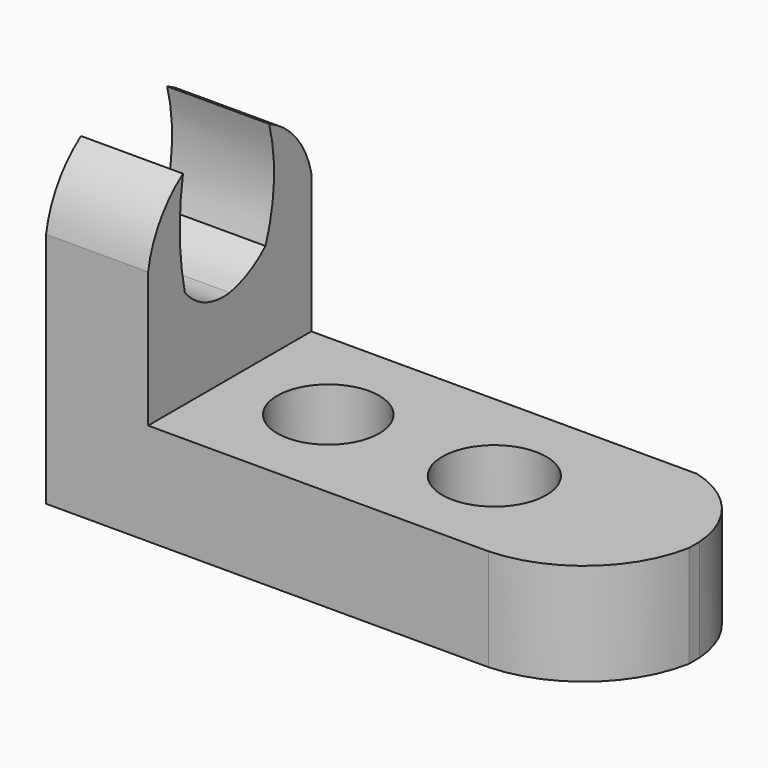
from build123d import *

# Parameters (mm, degrees)
F1_DEPTH = 25.4
F3_DEPTH = 25.4
F5_DEPTH = 25.4
F7_DEPTH = 25.4
F8_R     = 6.3524650116
F8_R_2   = 6.4782695501
F9_DEPTH = 25.4


with BuildPart() as f1:
    # F0 (on Front) → F1 (new body)
    with BuildSketch(Plane.XZ):
        Polygon((0, 38.1), (0, 0), (69.85, 0), (69.85, 12.7), (12.7, 12.7), (12.7, 38.1), align=None)
    extrude(amount=F1_DEPTH)

    # F2 (on face) → F3 (cut)
    with BuildSketch(Plane.XY.offset(12.7)):
        with BuildLine():
            ThreePointArc((69.85, -12.7), (64.6936030033, -21.620488158), (55.1082585024, -25.4))
            Line((55.1082585024, -25.4), (69.85, -25.4))
            Line((69.85, -25.4), (69.85, -12.7))
        make_face()
        with BuildLine():
            ThreePointArc((60.7121499118, 0), (67.063378566, -4.0558500097), (69.85, -11.0574759425))
            Line((69.85, -11.0574759425), (69.85, 0))
            Line((69.85, 0), (60.7121499118, 0))
        make_face()
    extrude(amount=-F3_DEPTH, mode=Mode.SUBTRACT)

    # F4 (on face) → F5 (cut)
    with BuildSketch(Plane.YZ.offset(12.7)):
        with BuildLine():
            ThreePointArc((-12.7, 22.1061483026), (-9.7123568594, 23.1357247682), (-7.1310154162, 24.958556518))
            ThreePointArc((-7.1310154162, 24.958556518), (-5.8144018077, 31.4845054838), (-6.5605342388, 38.1))
            Line((-6.5605342388, 38.1), (-19.9668444693, 38.1))
            ThreePointArc((-19.9668444693, 38.1), (-20.4652180352, 31.5153652578), (-19.6816045791, 24.958556518))
            ThreePointArc((-19.6816045791, 24.958556518), (-16.5691552263, 22.6062890993), (-12.7, 22.1061483026))
        make_face()
    extrude(amount=-F5_DEPTH, mode=Mode.SUBTRACT)

    # F6 (on face) → F7 (cut)
    with BuildSketch(Plane.YZ.offset(12.7)):
        with BuildLine():
            ThreePointArc((-25.4, 29.5361254617), (-23.5608826076, 34.3747475185), (-19.9668444693, 38.1))
            Line((-19.9668444693, 38.1), (-25.4, 38.1))
            Line((-25.4, 38.1), (-25.4, 29.5361254617))
        make_face()
        with BuildLine():
            Line((0, 38.1), (-6.5605342388, 38.1))
            ThreePointArc((-6.5605342388, 38.1), (-2.3318615541, 34.8502011083), (0, 30.0538183876))
            Line((0, 30.0538183876), (0, 38.1))
        make_face()
    extrude(amount=-F7_DEPTH, mode=Mode.SUBTRACT)

    # F8 (on face) → F9 (cut)
    with BuildSketch(Plane.XY.offset(12.7)):
        with Locations((24.9249059707, -12.6440813765)):
            Circle(F8_R)
        with Locations((45.6017628312, -12.6440813765)):
            Circle(F8_R_2)
    extrude(amount=-F9_DEPTH, mode=Mode.SUBTRACT)


solid = f1.part
